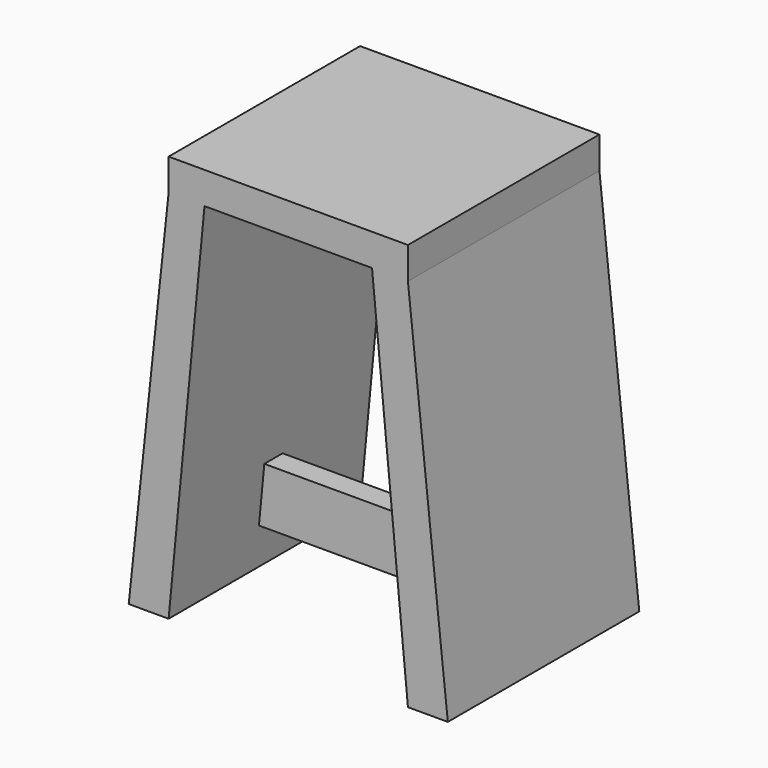
from build123d import *

# Parameters (mm, degrees)
F0_W          = 300
F0_H          = 300
F1_DEPTH      = 40
F4_W          = 45
F4_H          = 300
F3_W          = 50
F3_H          = 300
F7_W          = 28.6667700857
F7_H          = 70.264339447
F8_DEPTH      = 150
F8_DEPTH_BACK = 150


# Not quite as in the source:
# - an extrude ends at something that could not be found from the text; its depth is read off the source's solid


with BuildPart() as f1:
    # F0 (on Top) → F1 (new body)
    with BuildSketch(Plane.XY):
        Rectangle(F0_W, F0_H)
    extrude(amount=F1_DEPTH)

    # F4 (on face) → F5 section 0
    with BuildSketch(Plane(origin=(0, 0, 0), x_dir=(1, 0, 0), z_dir=(0, 0, -1))):
        with Locations((127.5, 0)):
            Rectangle(F4_W, F4_H)
    # F3 (on offset) → F5 section 1
    with BuildSketch(Plane(origin=(0, 0, -470), x_dir=(1, 0, 0), z_dir=(0, 0, -1))):
        with Locations((175, 0)):
            Rectangle(F3_W, F3_H)
    loft()

    # F6: F1 across plane


with BuildPart() as f1_1:
    add(f1.part)
    add(f1.part.mirror(Plane.YZ))

    # F7 (on Right) → F8 (join, two sides)
    with BuildSketch(Plane.YZ) as f8_sk:
        with Locations((0, -385.5957090855)):
            Rectangle(F7_W, F7_H)
    extrude(amount=F8_DEPTH)
    extrude(f8_sk.sketch, amount=-F8_DEPTH_BACK)


solid = f1_1.part
